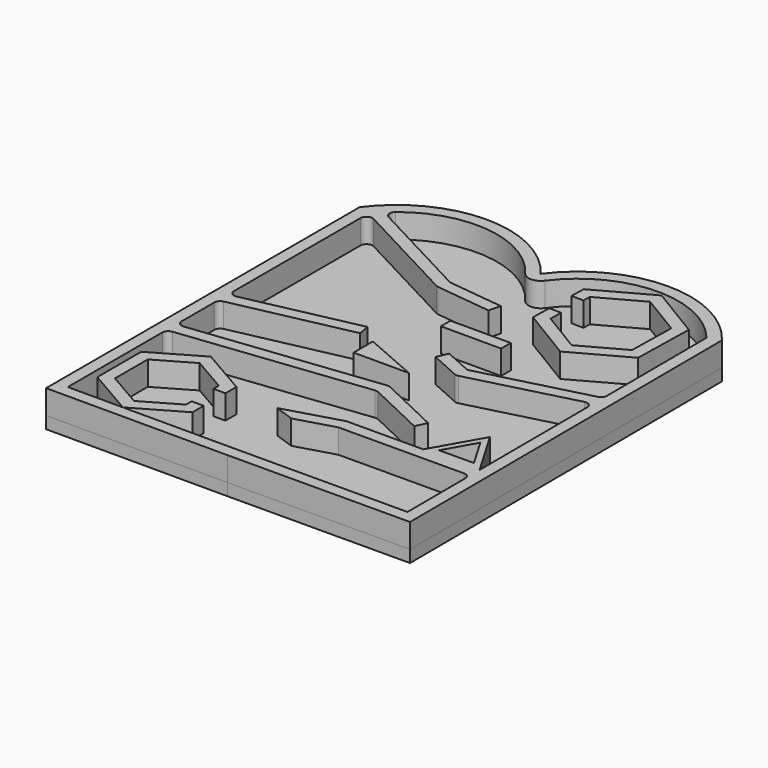
from build123d import *

# Parameters (mm, degrees)
F1_DEPTH = 6
F0_W     = 10
F0_H     = 2
F3_DEPTH = 2


# Not quite as in the source:
# - ends of sketch curves that miss each other by under 0.0002 mm in the source are joined


with BuildPart() as f1:
    # F0 (on Top) → F1 (new body)
    with BuildSketch(Plane.XY):
        with BuildLine():
            Line((-30, 32.3473930837), (-30, -32.6526069163))
            Line((-30, -32.6526069163), (0.1192900786, -32.6526069163))
            Line((0.1192900786, -32.6526069163), (30.2382853209, -32.5193386265))
            Line((30.2382853209, -32.5193386265), (29.9506809711, 32.4800250915))
            ThreePointArc((29.9506809711, 32.4800250915), (14.938018386, 39.9687184444), (-0.0245860478, 32.3805016191))
            ThreePointArc((-0.0245860478, 32.3805016191), (-15.0206194621, 39.9024393927), (-30, 32.3473930837))
        make_face()
        with BuildLine():
            Line((-18.8592523336, -30.6526069163), (-28, -30.6526069163))
            Line((-28, -30.6526069163), (-28, -11.0710615659))
            ThreePointArc((-28, -11.0710615659), (-27.7465009831, -10.4056772542), (-27.1145274354, -10.0776414803))
            Line((-27.1145274354, -10.0776414803), (3.6698389075, -6.5286347923))
            ThreePointArc((3.6698389075, -6.5286347923), (3.9474323278, -6.5354397125), (4.2124526409, -6.6183170169))
            Line((4.2124526409, -6.6183170169), (13.8885083595, -11.2017112184))
            Line((13.8885083595, -11.2017112184), (14.7446809555, -9.3942354963))
            Line((14.7446809555, -9.3942354963), (4.5516618753, -4.5659639457))
            ThreePointArc((4.5516618753, -4.5659639457), (4.2866415622, -4.4830866414), (4.0090481419, -4.4762817211))
            Line((4.0090481419, -4.4762817211), (-26.8854725646, -8.0379876659))
            ThreePointArc((-26.8854725646, -8.0379876659), (-27.6653843117, -7.7910685633), (-28, -7.0445675803))
            Line((-28, -7.0445675803), (-28, -0.3031208943))
            ThreePointArc((-28, -0.3031208943), (-27.777063149, 0.3263017478), (-27.2076542751, 0.6750813864))
            Line((-27.2076542751, 0.6750813864), (-7.8752691202, 4.7789896525))
            Line((-7.8752691202, 4.7789896525), (-8.2269339416, 6.748904602))
            Line((-8.2269339416, 6.748904602), (-26.7923457249, 2.8078106154))
            ThreePointArc((-26.7923457249, 2.8078106154), (-27.6294226421, 3.0089497471), (-28, 3.7860128961))
            Line((-28, 3.7860128961), (-28, 30.0059348114))
            ThreePointArc((-28, 30.0059348114), (-27.5159136269, 30.8625754184), (-26.5323337407, 30.8898399364))
            Line((-26.5323337407, 30.8898399364), (-8.4484836928, 21.3218373695))
            ThreePointArc((-8.4484836928, 21.3218373695), (-8.2777475055, 21.2508432682), (-8.0968589797, 21.212498134))
            Line((-8.0968589797, 21.212498134), (1.1104592122, 20.1367996633))
            Line((1.1104592122, 20.1367996633), (1.589740147, 22.0944080593))
            Line((1.589740147, 22.0944080593), (-7.4926699193, 23.1555134121))
            ThreePointArc((-7.4926699193, 23.1555134121), (-7.673558445, 23.1938585463), (-7.8442946323, 23.2648526476))
            Line((-7.8442946323, 23.2648526476), (-25.336579259, 32.5198632656))
            ThreePointArc((-25.336579259, 32.5198632656), (-25.864176528, 33.3065546609), (-25.4987813298, 34.1804703197))
            ThreePointArc((-25.4987813298, 34.1804703197), (-12.9378201369, 37.7743931473), (-1.6438298189, 31.2063028557))
            ThreePointArc((-1.6438298189, 31.2063028557), (-0.0201923897, 30.3945345597), (1.599837329, 31.2134789892))
            ThreePointArc((1.599837329, 31.2134789892), (14.6353510123, 37.9648321663), (27.9537138644, 31.790158276))
            Line((27.9537138644, 31.790158276), (28.0455327124, 11.0388493912))
            ThreePointArc((28.0455327124, 11.0388493912), (27.837893783, 10.4243595923), (27.2969034481, 10.0665312879))
            Line((27.2969034481, 10.0665312879), (9.7187459346, 5.5015014827))
            ThreePointArc((9.7187459346, 5.5015014827), (9.3831012246, 5.4729531105), (9.0570203938, 5.557473361))
            Line((9.0570203938, 5.557473361), (4.7224049972, 7.5080498132))
            Line((4.7224049972, 7.5080498132), (3.9016758092, 5.6842067279))
            Line((3.9016758092, 5.6842067279), (8.8783137321, 3.4447202094))
            ThreePointArc((8.8783137321, 3.4447202094), (9.2043945629, 3.3601999588), (9.5400392729, 3.388748331))
            Line((9.5400392729, 3.388748331), (26.8124465698, 7.8743751129))
            ThreePointArc((26.8124465698, 7.8743751129), (27.6738726331, 7.6988329735), (28.0637977276, 6.9109063742))
            Line((28.0637977276, 6.9109063742), (28.1629825794, -15.5051393439))
            Line((28.1629825794, -15.5051393439), (23.4331540021, -7.4645135844))
            Line((23.4331540021, -7.4645135844), (18.8542303832, -15.5463280182))
            Line((18.8542303832, -15.5463280182), (6.1433850081, -15.6025700214))
            Line((6.1433850081, -15.6025700214), (-3.1372315382, -18.3176588576))
            Line((-3.1372315382, -18.3176588576), (0.0900974588, -19.4573196774))
            Line((0.0900974588, -19.4573196774), (6.4342668447, -17.6013025272))
            Line((6.4342668447, -17.6013025272), (27.1718417329, -17.5095444483))
            ThreePointArc((27.1718417329, -17.5095444483), (27.8802375517, -17.7993060772), (28.1762566263, -18.5051099771))
            Line((28.1762566263, -18.5051099771), (28.2294555342, -30.528207569))
            Line((28.2294555342, -30.528207569), (0.1148653747, -30.6526069163))
            Line((0.1148653747, -30.6526069163), (-18.8592523336, -30.6526069163))
        make_face(mode=Mode.SUBTRACT)
        Polygon((20.6070848965, -14.4811387909), (23.4493978311, -9.4644476178), (26.3728233626, -14.4343084113), align=None, mode=Mode.SUBTRACT)
    extrude(amount=F1_DEPTH)


with BuildPart() as f1b:
    # F0 (on Top) → F1, piece 2 (new body)
    with BuildSketch(Plane.XY):
        Polygon((22.7288285259, 31.0075356756), (22.5648244879, 23.0787793067), (15.616318033, 19.2564327856), (8.8318156161, 23.3628426333), (8.8761979714, 25.5085024983), (6.8766256914, 25.549863074), (6.8083637966, 22.2497496149), (15.5685589539, 16.9475255974), (24.5405172283, 21.8829651369), (24.7522803454, 32.120628694), (15.9920851882, 37.4228527116), (7.0201269138, 32.487413172), (6.9696869869, 30.0489007039), (8.9692592668, 30.0075401282), (8.9958196542, 31.2915990022), (15.9443261091, 35.1139455234), align=None)
    extrude(amount=F1_DEPTH)


with BuildPart() as f1c:
    # F0 (on Top) → F1, piece 3 (new body)
    with BuildSketch(Plane.XY):
        with Locations((4.0708723292, 13.8201162443)):
            Rectangle(F0_W, F0_H)
    extrude(amount=F1_DEPTH)


with BuildPart() as f1d:
    # F0 (on Top) → F1, piece 4 (new body)
    with BuildSketch(Plane.XY):
        Polygon((-5.1392655546, 4), (-5.1392655546, 0), (4.0258858353, 0), align=None)
    extrude(amount=F1_DEPTH)


with BuildPart() as f1e:
    # F0 (on Top) → F1, piece 5 (new body)
    with BuildSketch(Plane.XY):
        Polygon((-26.7476101638, -26.0982613996), (-18.8592523336, -30.6526069163), (-10.9708945035, -26.0982613996), (-10.9708945035, -23.7670542747), (-12.9708945035, -23.7670542747), (-12.9708945035, -24.9435608612), (-18.8592523336, -28.3432058396), (-24.7476101638, -24.9435608612), (-24.7476101638, -18.1442709045), (-18.8592523336, -14.7446259262), (-12.9708945035, -18.1442709045), (-12.9708945035, -19.2670542747), (-10.9708945035, -19.2670542747), (-10.9708945035, -16.9895703661), (-18.8592523336, -12.4352248494), (-26.7476101638, -16.9895703661), align=None)
    extrude(amount=F1_DEPTH)


with BuildPart() as f3:
    # F2 (on Top) → F3 (new body)
    with BuildSketch(Plane.XY):
        with BuildLine():
            Line((-30, 32.3473930837), (-30, -32.6526069163))
            Line((-30, -32.6526069163), (0.1192900786, -32.6526069163))
            Line((0.1192900786, -32.6526069163), (30.2382853209, -32.5193386265))
            Line((30.2382853209, -32.5193386265), (29.9506809711, 32.4800250915))
            ThreePointArc((29.9506809711, 32.4800250915), (14.938018386, 39.9687184444), (-0.0245860478, 32.3805016191))
            ThreePointArc((-0.0245860478, 32.3805016191), (-15.0206194621, 39.9024393927), (-30, 32.3473930837))
        make_face()
    extrude(amount=F3_DEPTH)


solid = Compound([f1.part, f1b.part, f1c.part, f1d.part, f1e.part, f3.part])
